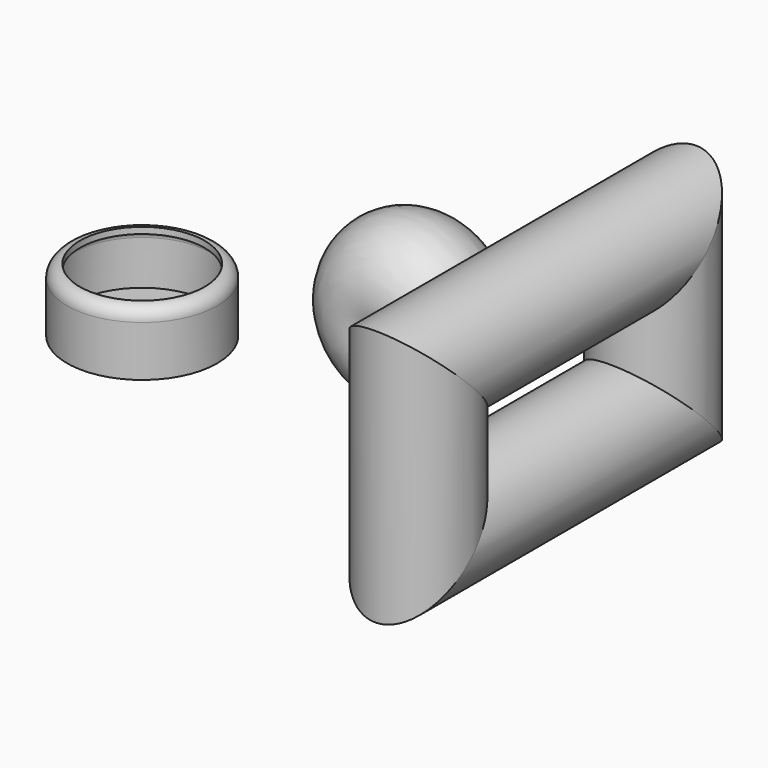
from build123d import *

# Parameters (mm, degrees)
F2_R     = 30.150829
F3_DEPTH = 25.4
F4_R     = 5.08
F5_T     = -2.54
F6_R     = 21.650929


# Not quite as in the source:
# - a shell that OpenCascade refuses in one call is made with other operations: the cavity is built on its own and cut out


with BuildPart() as f1:
    # F0 (on Top) → F1 (revolve)
    with BuildSketch(Plane.XY):
        with BuildLine():
            Line((0, 41.393153), (0, 0))
            ThreePointArc((0, 0), (33.348054, 20.696577), (0, 41.393153))
        make_face()
    revolve(axis=Axis((0, 20.696577, 0), (0, 1, 0)))


with BuildPart() as f3:
    # F2 (on Top) → F3 (new body)
    with BuildSketch(Plane.XY):
        with Locations((-54.787904, -46.353389)):
            Circle(F2_R)
    extrude(amount=F3_DEPTH)

    # F4
    f4_edges = [f3.edges().sort_by_distance(p)[0] for p in [
        (-84.938733, -46.353389, 25.4),
    ]]
    fillet(f4_edges, radius=F4_R)

    # F5: a shell. OpenCascade refuses it in one call, so the cavity is built on its own and cut out:
    # the body offset inwards by the wall thickness, plus a prism from it out through each open face.
    f5_core = offset(f3.part, amount=F5_T, mode=Mode.PRIVATE)
    f5_exits = [f5_core.faces().sort_by_distance(p)[0] for p in [
        (-54.787904, -46.353389, 22.86),
    ]]
    add(f5_core, mode=Mode.SUBTRACT)
    extrude(f5_exits, amount=-F5_T, mode=Mode.SUBTRACT)


with BuildPart() as f9:
    # F9: sweep along a path in F8
    with BuildLine(Plane.YZ.offset(97.510114)) as f9_path:
        Line((19.326866, 0), (19.326866, 59.012301))
        Line((19.326866, 59.012301), (-97.731575, 59.012301))
        Line((-97.731575, 59.012301), (-97.731575, 0))
        Line((-97.731575, 0), (19.326866, 0))
    # F6 (on Top) → F9 (sweep)
    with BuildSketch(Plane.XY):
        with Locations((97.510114, 19.718664)):
            Circle(F6_R)
    sweep(path=f9_path.line, transition=Transition.RIGHT)


solid = Compound([f1.part, f3.part, f9.part])
